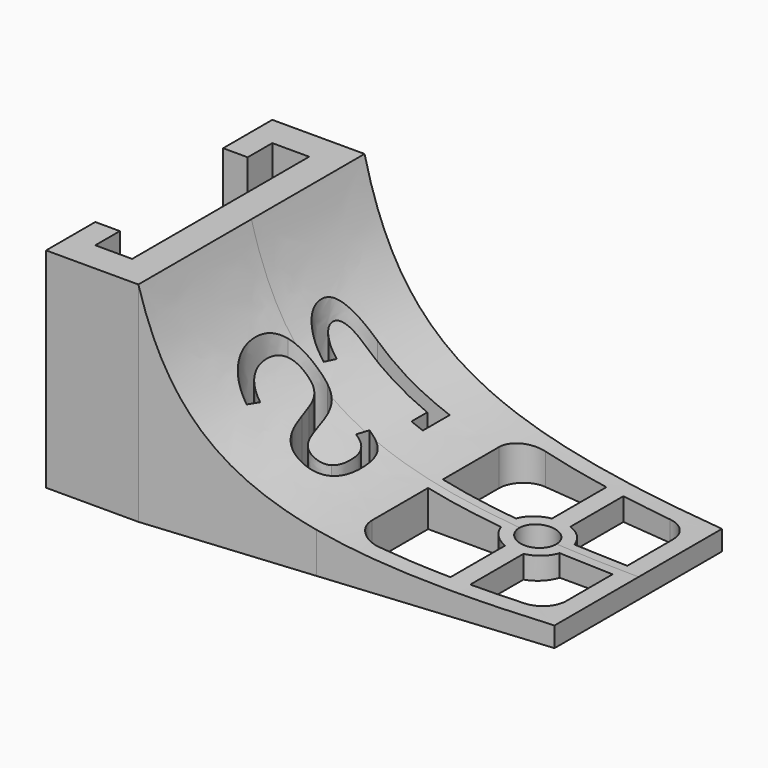
from build123d import *

# Parameters (mm, degrees)
F1_DEPTH      = 17
F2_R          = 1.5
F3_DEPTH      = 17
F5_DEPTH      = 25
F5_DEPTH_BACK = 25
F6_R          = 2


with BuildPart() as f1:
    # F0 (on Top) → F1 (new body)
    with BuildSketch(Plane.XY):
        Polygon((-1, 9), (-1, -9), (-4, -9), (-4, -6.5), (-6, -6.5), (-6, -11.5), (1.5, -11.5), (1.5, 11.5), (-6, 11.5), (-6, 6.5), (-4, 6.5), (-4, 9), align=None)
    extrude(amount=F1_DEPTH)

    # F2 (on face) → F3 (join)
    with BuildSketch(Plane(origin=(0, 0, 0), x_dir=(1, 0, 0), z_dir=(0, 0, -1))):
        Polygon((15, -10.2009244547), (15, 10.2383274636), (1.5, 11.5), (1.5, -11.5), align=None)
        with BuildLine():
            add(Edge.make_bspline(
                [(4.835088208, -5.6240248599), (4.1383223358, -4.9661261996), (4.1383223358, -3.8228613807)],
                knots=[0, 0, 0, 1, 1, 1], degree=2))
            add(Edge.make_bspline(
                [(4.1383223358, -3.8228613807), (4.1383223358, -1.7012803984), (6.3319498573, -1.3050244329)],
                knots=[0, 0, 0, 1, 1, 1], degree=2))
            Line((6.3319498573, -1.3050244329), (6.5158581283, -2.4122659823))
            add(Edge.make_bspline(
                [(6.5158581283, -2.4122659823), (5.8276240831, -2.520335791), (5.442743887, -2.892892237)],
                knots=[0, 0, 0, 1, 1, 1], degree=2))
            add(Edge.make_bspline(
                [(5.442743887, -2.892892237), (5.0578636909, -3.2654486829), (5.0578636909, -3.8285492654)],
                knots=[0, 0, 0, 1, 1, 1], degree=2))
            add(Edge.make_bspline(
                [(5.0578636909, -3.8285492654), (5.0578636909, -4.4447367714), (5.4816110989, -4.8002295633)],
                knots=[0, 0, 0, 1, 1, 1], degree=2))
            add(Edge.make_bspline(
                [(5.4816110989, -4.8002295633), (5.9053585069, -5.1557223553), (6.722517938, -5.1557223553)],
                knots=[0, 0, 0, 1, 1, 1], degree=2))
            Line((6.722517938, -5.1557223553), (11.6823533712, -5.1557223553))
            Line((11.6823533712, -5.1557223553), (11.6823533712, -3.5498429165))
            Line((11.6823533712, -3.5498429165), (12.6056866495, -3.5498429165))
            Line((12.6056866495, -3.5498429165), (12.6056866495, -6.2819235202))
            Line((12.6056866495, -6.2819235202), (6.7471654383, -6.2819235202))
            add(Edge.make_bspline(
                [(6.7471654383, -6.2819235202), (5.5318540802, -6.2819235202), (4.835088208, -5.6240248599)],
                knots=[0, 0, 0, 1, 1, 1], degree=2))
        make_face(mode=Mode.SUBTRACT)
        with BuildLine():
            add(Edge.make_bspline(
                [(7.3567170788, -0.4309861551), (7.0182879409, -0.5580155795), (6.5632571672, -0.5580155795)],
                knots=[0, 0, 0, 1, 1, 1], degree=2))
            add(Edge.make_bspline(
                [(6.5632571672, -0.5580155795), (5.4067206174, -0.5580155795), (4.7725214766, 0.3454101025)],
                knots=[0, 0, 0, 1, 1, 1], degree=2))
            add(Edge.make_bspline(
                [(4.7725214766, 0.3454101025), (4.1383223358, 1.2488357844), (4.1383223358, 2.8907384928)],
                knots=[0, 0, 0, 1, 1, 1], degree=2))
            add(Edge.make_bspline(
                [(4.1383223358, 2.8907384928), (4.1383223358, 5.941340638), (6.2599033181, 6.4267067967)],
                knots=[0, 0, 0, 1, 1, 1], degree=2))
            Line((6.2599033181, 6.4267067967), (6.4798348587, 5.3308410167))
            add(Edge.make_bspline(
                [(6.4798348587, 5.3308410167), (5.7271381206, 5.141244861), (5.374489271, 4.5250573549)],
                knots=[0, 0, 0, 1, 1, 1], degree=2))
            add(Edge.make_bspline(
                [(5.374489271, 4.5250573549), (5.0218404213, 3.9088698489), (5.0218404213, 2.8490273385)],
                knots=[0, 0, 0, 1, 1, 1], degree=2))
            add(Edge.make_bspline(
                [(5.0218404213, 2.8490273385), (5.0218404213, 1.7531615586), (5.3981887904, 1.1578296296)],
                knots=[0, 0, 0, 1, 1, 1], degree=2))
            add(Edge.make_bspline(
                [(5.3981887904, 1.1578296296), (5.7745371595, 0.5624977007), (6.5025863974, 0.5624977007)],
                knots=[0, 0, 0, 1, 1, 1], degree=2))
            add(Edge.make_bspline(
                [(6.5025863974, 0.5624977007), (6.9121140937, 0.5624977007), (7.1671209231, 0.7483019333)],
                knots=[0, 0, 0, 1, 1, 1], degree=2))
            add(Edge.make_bspline(
                [(7.1671209231, 0.7483019333), (7.4221277526, 0.9341061659), (7.5880243888, 1.2725353038)],
                knots=[0, 0, 0, 1, 1, 1], degree=2))
            add(Edge.make_bspline(
                [(7.5880243888, 1.2725353038), (7.753921025, 1.6109644418), (7.8667307377, 2.0783189656)],
                knots=[0, 0, 0, 1, 1, 1], degree=2))
            add(Edge.make_bspline(
                [(7.8667307377, 2.0783189656), (7.9795404503, 2.5456734894), (8.1084658362, 3.1144619565)],
                knots=[0, 0, 0, 1, 1, 1], degree=2))
            add(Edge.make_bspline(
                [(8.1084658362, 3.1144619565), (8.3283973768, 4.1041538893), (8.5473809367, 4.6170114905)],
                knots=[0, 0, 0, 1, 1, 1], degree=2))
            add(Edge.make_bspline(
                [(8.5473809367, 4.6170114905), (8.7663644965, 5.1298690916), (9.0365390184, 5.4256390945)],
                knots=[0, 0, 0, 1, 1, 1], degree=2))
            add(Edge.make_bspline(
                [(9.0365390184, 5.4256390945), (9.3067135403, 5.7214090974), (9.6678942169, 5.8787739067)],
                knots=[0, 0, 0, 1, 1, 1], degree=2))
            add(Edge.make_bspline(
                [(9.6678942169, 5.8787739067), (10.0290748935, 6.0361387159), (10.4973773981, 6.0361387159)],
                knots=[0, 0, 0, 1, 1, 1], degree=2))
            add(Edge.make_bspline(
                [(10.4973773981, 6.0361387159), (11.5685956778, 6.0361387159), (12.149707895, 5.2151873617)],
                knots=[0, 0, 0, 1, 1, 1], degree=2))
            add(Edge.make_bspline(
                [(12.149707895, 5.2151873617), (12.7308201123, 4.3942360075), (12.7308201123, 2.8660909925)],
                knots=[0, 0, 0, 1, 1, 1], degree=2))
            add(Edge.make_bspline(
                [(12.7308201123, 2.8660909925), (12.7308201123, 1.4441198248), (12.2947489541, 0.6914230866)],
                knots=[0, 0, 0, 1, 1, 1], degree=2))
            add(Edge.make_bspline(
                [(12.2947489541, 0.6914230866), (11.858677796, -0.0612736515), (10.810211055, -0.3627315391)],
                knots=[0, 0, 0, 1, 1, 1], degree=2))
            Line((10.810211055, -0.3627315391), (10.6149270146, 0.7520938564))
            add(Edge.make_bspline(
                [(10.6149270146, 0.7520938564), (11.2785135596, 0.9341061659), (11.5780754856, 1.4498077094)],
                knots=[0, 0, 0, 1, 1, 1], degree=2))
            add(Edge.make_bspline(
                [(11.5780754856, 1.4498077094), (11.8776374116, 1.9655092529), (11.8776374116, 2.8774667619)],
                knots=[0, 0, 0, 1, 1, 1], degree=2))
            add(Edge.make_bspline(
                [(11.8776374116, 2.8774667619), (11.8776374116, 3.8804304256), (11.5458441391, 4.4075077384)],
                knots=[0, 0, 0, 1, 1, 1], degree=2))
            add(Edge.make_bspline(
                [(11.5458441391, 4.4075077384), (11.2140508666, 4.9345850513), (10.5561522063, 4.9345850513)],
                knots=[0, 0, 0, 1, 1, 1], degree=2))
            add(Edge.make_bspline(
                [(10.5561522063, 4.9345850513), (10.1712720103, 4.9345850513), (9.9191091232, 4.7298212031)],
                knots=[0, 0, 0, 1, 1, 1], degree=2))
            add(Edge.make_bspline(
                [(9.9191091232, 4.7298212031), (9.6669462361, 4.5250573549), (9.4925177728, 4.1401771589)],
                knots=[0, 0, 0, 1, 1, 1], degree=2))
            add(Edge.make_bspline(
                [(9.4925177728, 4.1401771589), (9.3180893096, 3.7552969628), (9.0621344994, 2.6063442592)],
                knots=[0, 0, 0, 1, 1, 1], degree=2))
            add(Edge.make_bspline(
                [(9.0621344994, 2.6063442592), (8.9749202678, 2.2214640631), (8.8829661323, 1.8384798286)],
                knots=[0, 0, 0, 1, 1, 1], degree=2))
            add(Edge.make_bspline(
                [(8.8829661323, 1.8384798286), (8.7910119967, 1.4554955941), (8.6630345916, 1.1066386676)],
                knots=[0, 0, 0, 1, 1, 1], degree=2))
            add(Edge.make_bspline(
                [(8.6630345916, 1.1066386676), (8.5350571865, 0.7577817411), (8.3634726656, 0.4525319304)],
                knots=[0, 0, 0, 1, 1, 1], degree=2))
            add(Edge.make_bspline(
                [(8.3634726656, 0.4525319304), (8.1918881447, 0.1472821197), (7.9435171807, -0.0783373055)],
                knots=[0, 0, 0, 1, 1, 1], degree=2))
            add(Edge.make_bspline(
                [(7.9435171807, -0.0783373055), (7.6951462168, -0.3039567308), (7.3567170788, -0.4309861551)],
                knots=[0, 0, 0, 1, 1, 1], degree=2))
        make_face(mode=Mode.SUBTRACT)
        Polygon((33, 8.5560974151), (15, 10.2383274636), (15, -10.2009244547), (33, -8.4688237275), align=None)
        Polygon((31.5, 7.2775398239), (31.5, 0.7823054263), (31.5, -0.7176945737), (31.5, -7.1713700725), (25.5702230149, -7.741979574), (24.0702230149, -7.8863213012), (16.5, -8.6147873451), (16.5, -0.7176945737), (16.5, 0.7823054263), (16.5, 8.6793981977), (24.0702230149, 7.9719061627), (25.5702230149, 7.8317203253), align=None, mode=Mode.SUBTRACT)
        with BuildLine():
            ThreePointArc((22.4353750114, -0.7176945737), (22.3202230149, 0.0323054263), (22.4353750114, 0.7823054263))
            Line((22.4353750114, 0.7823054263), (16.5, 0.7823054263))
            Line((16.5, 0.7823054263), (16.5, -0.7176945737))
            Line((16.5, -0.7176945737), (22.4353750114, -0.7176945737))
        make_face()
        with BuildLine():
            Line((25.5702230149, -7.741979574), (25.5702230149, -2.3525425772))
            ThreePointArc((25.5702230149, -2.3525425772), (24.8202230149, -2.4676945737), (24.0702230149, -2.3525425772))
            Line((24.0702230149, -2.3525425772), (24.0702230149, -7.8863213012))
            Line((24.0702230149, -7.8863213012), (25.5702230149, -7.741979574))
        make_face()
        with BuildLine():
            ThreePointArc((27.2050710185, 0.7823054263), (27.2912673295, 0.4116996745), (27.3202230149, 0.0323054263))
            ThreePointArc((27.3202230149, 0.0323054263), (27.2912673295, -0.3470888219), (27.2050710185, -0.7176945737))
            Line((27.2050710185, -0.7176945737), (31.5, -0.7176945737))
            Line((31.5, -0.7176945737), (31.5, 0.7823054263))
            Line((31.5, 0.7823054263), (27.2050710185, 0.7823054263))
        make_face()
        with BuildLine():
            ThreePointArc((24.0702230149, 2.4171534299), (24.8202230149, 2.5323054263), (25.5702230149, 2.4171534299))
            Line((25.5702230149, 2.4171534299), (25.5702230149, 7.8317203253))
            Line((25.5702230149, 7.8317203253), (24.0702230149, 7.9719061627))
            Line((24.0702230149, 7.9719061627), (24.0702230149, 2.4171534299))
        make_face()
        with BuildLine():
            ThreePointArc((27.2050710185, -0.7176945737), (27.2912673295, -0.3470888219), (27.3202230149, 0.0323054263))
            ThreePointArc((27.3202230149, 0.0323054263), (27.2912673295, 0.4116996745), (27.2050710185, 0.7823054263))
            ThreePointArc((27.2050710185, 0.7823054263), (26.5879899679, 1.8000723793), (25.5702230149, 2.4171534299))
            ThreePointArc((25.5702230149, 2.4171534299), (24.8202230149, 2.5323054263), (24.0702230149, 2.4171534299))
            ThreePointArc((24.0702230149, 2.4171534299), (23.052456062, 1.8000723793), (22.4353750114, 0.7823054263))
            ThreePointArc((22.4353750114, 0.7823054263), (22.3202230149, 0.0323054263), (22.4353750114, -0.7176945737))
            ThreePointArc((22.4353750114, -0.7176945737), (23.052456062, -1.7354615267), (24.0702230149, -2.3525425772))
            ThreePointArc((24.0702230149, -2.3525425772), (24.8202230149, -2.4676945737), (25.5702230149, -2.3525425772))
            ThreePointArc((25.5702230149, -2.3525425772), (26.5879899679, -1.7354615267), (27.2050710185, -0.7176945737))
        make_face()
        with Locations((24.8202230149, 0.0323054263)):
            Circle(F2_R, mode=Mode.SUBTRACT)
    extrude(amount=-F3_DEPTH)

    # F4 (on Front) → F5 (cut, two sides)
    with BuildSketch(Plane.XZ) as f5_sk:
        with BuildLine():
            add(Edge.make_bspline(
                [(33.1036038697, 1.6239841934), (12.0637770742, 1.7651917879), (4.5752389124, 4.9196225591), (1.3980838703, 17.4164324999)],
                knots=[0, 0, 0, 0, 35.4209178586, 35.4209178586, 35.4209178586, 35.4209178586], degree=3))
            Line((33.1036038697, 1.6239841934), (37.6334600151, 20.9869686514))
            Line((37.6334600151, 20.9869686514), (1.3980838703, 17.4164324999))
        make_face()
    extrude(amount=-F5_DEPTH, mode=Mode.SUBTRACT)
    extrude(f5_sk.sketch, amount=F5_DEPTH_BACK, mode=Mode.SUBTRACT)

    # F6
    f6_edges = [f1.edges().sort_by_distance(p)[0] for p in [
        (31.5, -7.27754, 0.820535),
        (31.5, 7.17137, 0.820535),
        (16.5, 8.614787, 1.473888),
        (16.5, -8.679398, 1.473888),
    ]]
    fillet(f6_edges, radius=F6_R)


solid = f1.part
